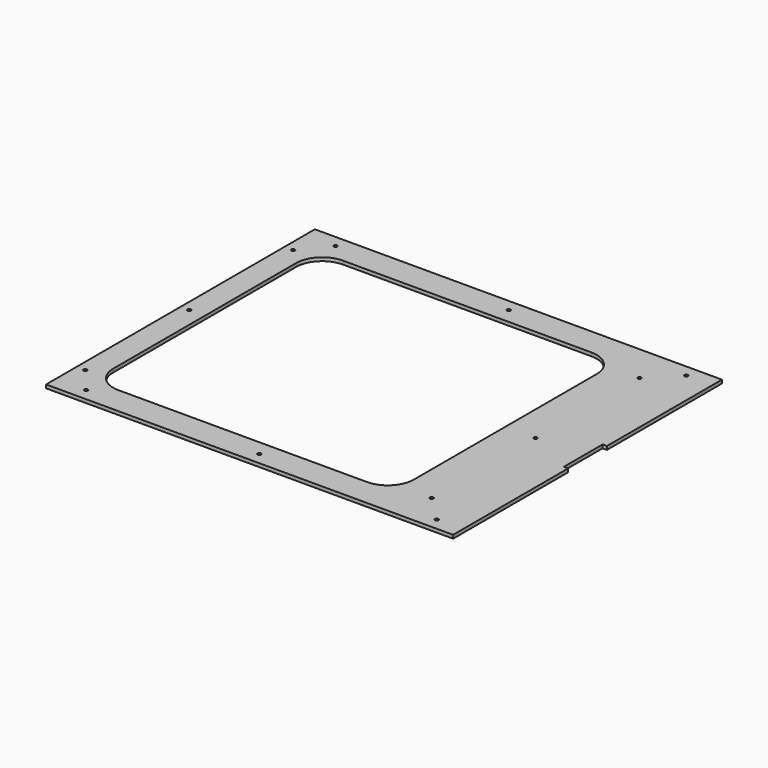
from build123d import *

# Parameters (mm, degrees)
F0_R     = 2
F1_DEPTH = 4


# Not quite as in the source:
# - a feature names something its author has since deleted; it is built from what else it names


with BuildPart() as f1:
    # F0 (on Top) → F1 (new body)
    with BuildSketch(Plane.XY):
        Polygon((-235, 194), (-235, 190), (-235, -170), (-235, -190), (-235, -194), (235, -194), (235, -190), (235, -28), (230, -28), (230, 0), (230, 28), (235, 28), (235, 190), (235, 194), align=None)
        with Locations((-200, -180)):
            Circle(F0_R, mode=Mode.SUBTRACT)
        with Locations((-225, -150)):
            Circle(F0_R, mode=Mode.SUBTRACT)
        with Locations((-225, 0)):
            Circle(F0_R, mode=Mode.SUBTRACT)
        with BuildLine():
            Line((110, -161.9999999998), (-177, -162))
            ThreePointArc((-177, -162), (-198.2132034356, -153.2132034356), (-207, -132))
            Line((-207, -132), (-207, 0))
            Line((-207, 0), (-207, 132))
            ThreePointArc((-207, 132), (-198.2132034356, 153.2132034356), (-177, 162))
            Line((-177, 162), (110, 161.9999999998))
            ThreePointArc((110, 161.9999999998), (131.2132034356, 153.2132034354), (140, 131.9999999998))
            Line((140, 131.9999999998), (140, 0))
            Line((140, 0), (140, -131.9999999998))
            ThreePointArc((140, -131.9999999998), (131.2132034356, -153.2132034354), (110, -161.9999999998))
        make_face(mode=Mode.SUBTRACT)
        with Locations((0, -180)):
            Circle(F0_R, mode=Mode.SUBTRACT)
        with Locations((175, -150)):
            Circle(F0_R, mode=Mode.SUBTRACT)
        with Locations((205, -180)):
            Circle(F0_R, mode=Mode.SUBTRACT)
        with Locations((175, 0)):
            Circle(F0_R, mode=Mode.SUBTRACT)
        with Locations((-225, 150)):
            Circle(F0_R, mode=Mode.SUBTRACT)
        with Locations((-200, 180)):
            Circle(F0_R, mode=Mode.SUBTRACT)
        with Locations((0, 180)):
            Circle(F0_R, mode=Mode.SUBTRACT)
        with Locations((175, 150)):
            Circle(F0_R, mode=Mode.SUBTRACT)
        with Locations((205, 180)):
            Circle(F0_R, mode=Mode.SUBTRACT)
    extrude(amount=F1_DEPTH)


solid = f1.part
